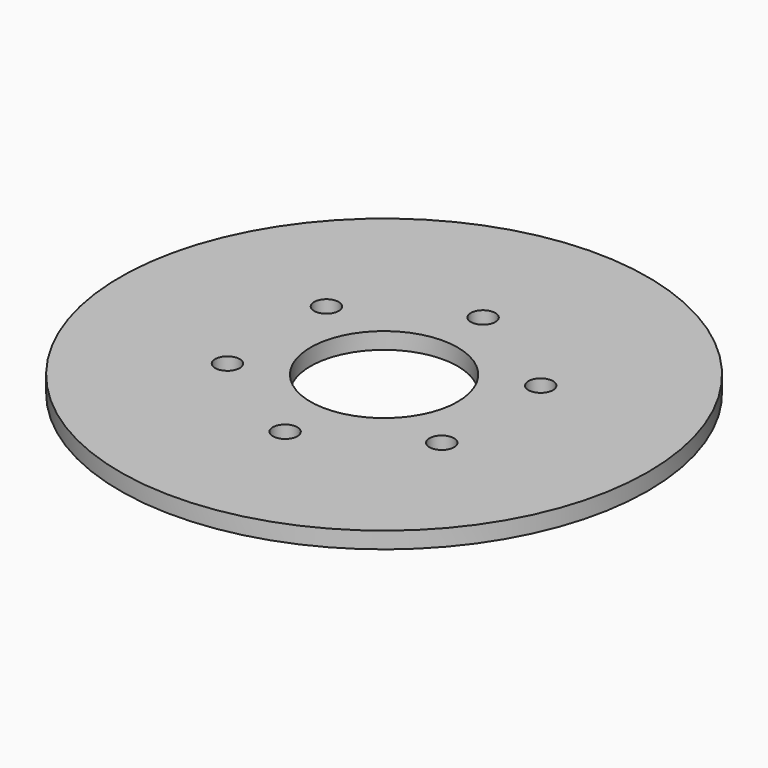
from build123d import *

# Parameters (mm, degrees)
F0_R            = 50.8
F0_R_2          = 14.1605
F1_DEPTH        = 3.175
F2_R            = 2.3622
F3_DEPTH        = 3.176
F3_COPIES_COUNT = 6


# Not quite as in the source:
# - a pattern or mirror of a feature is missing from the dataset's text; its kind, count and spacing are read off the source's solid


with BuildPart() as f1:
    # F0 (on Top) → F1 (new body)
    with BuildSketch(Plane.XY):
        Circle(F0_R)
        Circle(F0_R_2, mode=Mode.SUBTRACT)
    extrude(amount=F1_DEPTH)

    # F2 (on face) → F3 (cut, through all)
    with BuildSketch(Plane.XY.offset(3.175)):
        with Locations((0, 23.8125)):
            Circle(F2_R)
    f3 = extrude(amount=-F3_DEPTH, mode=Mode.SUBTRACT)

    # F3_copies: F3 ×6 about axis
    f3_copies_axis = Axis((0, 0, 0), (0, 0, 1))
    for i in range(1, F3_COPIES_COUNT):
        add(f3.rotate(f3_copies_axis, i * 360 / F3_COPIES_COUNT), mode=Mode.SUBTRACT)


solid = f1.part
